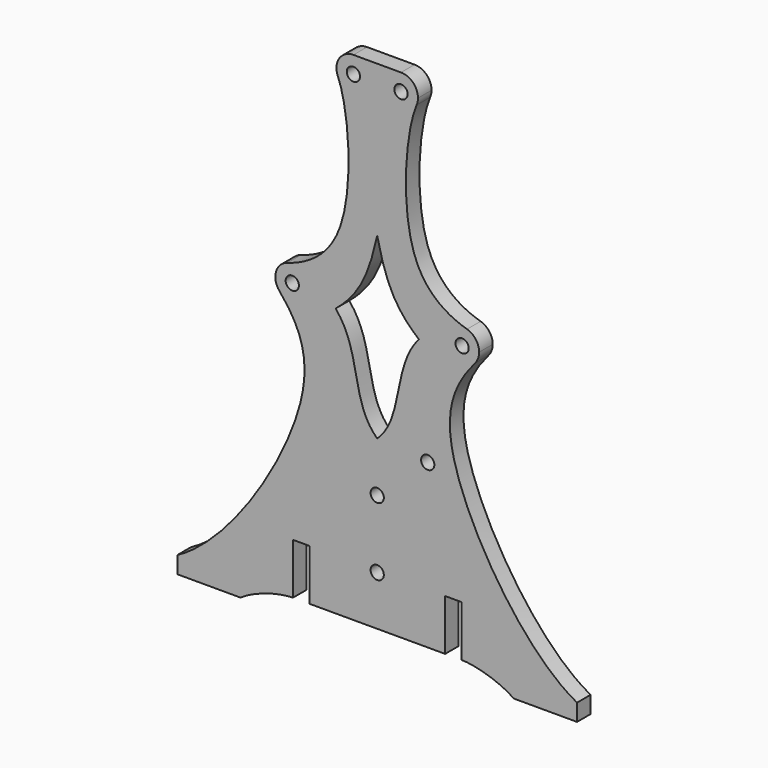
from build123d import *

# Parameters (mm, degrees)
F0_R     = 1.95
F1_DEPTH = 5


with BuildPart() as f1:
    # F0 (on Front) → F1 (new body)
    with BuildSketch(Plane.XZ):
        with BuildLine():
            ThreePointArc((11.5969807084, 58.0333357261), (11.8982090371, 58.9962329808), (12, 60))
            ThreePointArc((12, 60), (10.5355339059, 63.5355339059), (7, 65))
            ThreePointArc((7, 65), (2.8266727082, 57.2462136402), (11.5969807084, 58.0333357261))
        make_face()
        with Locations((7, 60)):
            Circle(F0_R, mode=Mode.SUBTRACT)
        with BuildLine():
            ThreePointArc((11.5969807084, 58.0333357261), (2.8266727082, 57.2462136402), (7, 65))
            Line((7, 65), (0, 65))
            Line((0, 65), (-7, 65))
            ThreePointArc((-7, 65), (-3.4644660941, 63.5355339059), (-2, 60))
            ThreePointArc((-2, 60), (-5.9962329808, 55.1017909629), (-11.5969807084, 58.0333357261))
            add(Edge.make_bspline(
                [(-11.5969807084, 58.0333357261), (-8.259178384, 50.2313874739), (-5.7002681923, 15.299773588), (-20.5659226075, 6.5540384245), (-26.4394786751, 4.7883087979)],
                knots=[0, 0, 0, 0, 0.5815539161, 1, 1, 1, 1], degree=3))
            ThreePointArc((-26.4394786751, 4.7883087979), (-22.0164947943, 4.0123181189), (-20, 0))
            ThreePointArc((-20, 0), (-23.271638205, -4.69177637), (-28.8051062023, -3.2436348113))
            add(Edge.make_bspline(
                [(-28.8051062023, -3.2436348113), (-22.7247010924, -10.376554681), (-15.2262960098, -29.050287314), (-43.232798529, -73.227558015), (-58.8278773565, -81.4663794637)],
                knots=[0, 0, 0, 0, 0.3913654049, 1, 1, 1, 1], degree=3))
            Line((-58.8278773565, -81.4663794637), (-58.8278773565, -86.4663794637))
            Line((-58.8278773565, -86.4663794637), (-40.2264967561, -86.4663794637))
            add(Edge.make_bspline(
                [(-24.8, -81.4663794637), (-27.8363596976, -81.4270702004), (-35.2759175003, -83.0063000321), (-40.2264967561, -86.4663794637)],
                knots=[0, 0, 0, 0, 16.2165595046, 16.2165595046, 16.2165595046, 16.2165595046], degree=3))
            Line((-24.8, -81.4663794637), (-24.8, -66.4663794637))
            Line((-24.8, -66.4663794637), (-20, -66.4663794637))
            Line((-20, -66.4663794637), (-20, -81.4663794637))
            Line((-20, -81.4663794637), (0, -81.4663794637))
            Line((0, -81.4663794637), (20, -81.4663794637))
            Line((20, -81.4663794637), (20, -66.4663794637))
            Line((20, -66.4663794637), (24.8, -66.4663794637))
            Line((24.8, -66.4663794637), (24.8, -81.4663794637))
            add(Edge.make_bspline(
                [(24.8, -81.4663794637), (27.8363596976, -81.4270702004), (35.2759175003, -83.0063000321), (40.2264967561, -86.4663794637)],
                knots=[0, 0, 0, 0, 16.2165595046, 16.2165595046, 16.2165595046, 16.2165595046], degree=3))
            Line((40.2264967561, -86.4663794637), (58.8278773565, -86.4663794637))
            Line((58.8278773565, -86.4663794637), (58.8278773565, -81.4663794637))
            add(Edge.make_bspline(
                [(28.8051062023, -3.2436348113), (22.7247010924, -10.376554681), (15.2262960098, -29.050287314), (43.232798529, -73.227558015), (58.8278773565, -81.4663794637)],
                knots=[0, 0, 0, 0, 0.3913654049, 1, 1, 1, 1], degree=3))
            ThreePointArc((28.8051062023, -3.2436348113), (20.2037048496, -1.4126403755), (26.4394786751, 4.7883087979))
            add(Edge.make_bspline(
                [(11.5969807084, 58.0333357261), (8.259178384, 50.2313874739), (5.7002681923, 15.299773588), (20.5659226075, 6.5540384245), (26.4394786751, 4.7883087979)],
                knots=[0, 0, 0, 0, 0.5815539161, 1, 1, 1, 1], degree=3))
        make_face()
        with Locations((0, -66.8700714409)):
            Circle(F0_R, mode=Mode.SUBTRACT)
        with Locations((0, -46.8700714409)):
            Circle(F0_R, mode=Mode.SUBTRACT)
        with Locations((14.8781873236, -33.5044610186)):
            Circle(F0_R, mode=Mode.SUBTRACT)
        with BuildLine():
            add(Edge.make_bspline(
                [(0, 20.4110946506), (-2.5965298992, 8.6431102827), (-5.6864479557, 2.9892178718), (-12.2460462153, -2.4297779892)],
                knots=[0, 0, 0, 0, 25.9166184302, 25.9166184302, 25.9166184302, 25.9166184302], degree=3))
            add(Edge.make_bspline(
                [(0, 20.4110946506), (2.5965298992, 8.6431102827), (5.6864479557, 2.9892178718), (12.2460462153, -2.4297779892)],
                knots=[0, 0, 0, 0, 25.9166184302, 25.9166184302, 25.9166184302, 25.9166184302], degree=3))
            add(Edge.make_bspline(
                [(12.2460462153, -2.4297779892), (4.406365566, -11.6358492523), (7.9564843327, -24.7844345868), (0, -32.1476459503)],
                knots=[0, 0, 0, 0, 32.1421424934, 32.1421424934, 32.1421424934, 32.1421424934], degree=3))
            add(Edge.make_bspline(
                [(-12.2460462153, -2.4297779892), (-4.406365566, -11.6358492523), (-7.9564843327, -24.7844345868), (0, -32.1476459503)],
                knots=[0, 0, 0, 0, 32.1421424934, 32.1421424934, 32.1421424934, 32.1421424934], degree=3))
        make_face(mode=Mode.SUBTRACT)
        with BuildLine():
            ThreePointArc((30, 0), (29.0123181189, 2.9835052057), (26.4394786751, 4.7883087979))
            ThreePointArc((26.4394786751, 4.7883087979), (20.2037048496, -1.4126403755), (28.8051062023, -3.2436348113))
            ThreePointArc((28.8051062023, -3.2436348113), (29.69177637, -1.728361795), (30, 0))
        make_face()
        with Locations((25, 0)):
            Circle(F0_R, mode=Mode.SUBTRACT)
        with BuildLine():
            ThreePointArc((-2, 60), (-3.4644660941, 63.5355339059), (-7, 65))
            ThreePointArc((-7, 65), (-11.1733272918, 62.7537863598), (-11.5969807084, 58.0333357261))
            ThreePointArc((-11.5969807084, 58.0333357261), (-5.9962329808, 55.1017909629), (-2, 60))
        make_face()
        with Locations((-7, 60)):
            Circle(F0_R, mode=Mode.SUBTRACT)
        with BuildLine():
            ThreePointArc((-20, 0), (-22.0164947943, 4.0123181189), (-26.4394786751, 4.7883087979))
            ThreePointArc((-26.4394786751, 4.7883087979), (-29.7962951504, 1.4126403755), (-28.8051062023, -3.2436348113))
            ThreePointArc((-28.8051062023, -3.2436348113), (-23.271638205, -4.69177637), (-20, 0))
        make_face()
        with Locations((-25, 0)):
            Circle(F0_R, mode=Mode.SUBTRACT)
    extrude(amount=F1_DEPTH)


solid = f1.part
